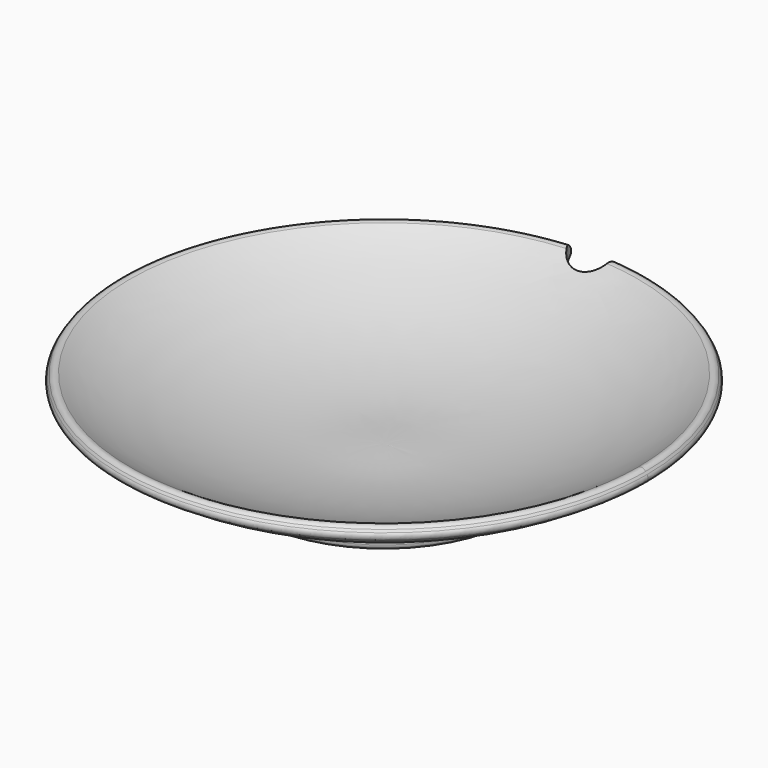
from build123d import *

# Parameters (mm, degrees)
F2_R     = 11.1276169932
F3_DEPTH = 87.884
F4_R     = 64.6620643292
F4_R_2   = 55.3121936168
F5_DEPTH = 5.334
F6_R     = 2.54


# Not quite as in the source:
# - ends of sketch curves that miss each other by under 0.0002 mm in the source are joined
# - the dataset's text gives a spline's control points without its knots; the knots are read off the source's solid


with BuildPart() as f1:
    # F0 (on Front) → F1 (revolve)
    with BuildSketch(Plane.XZ):
        with BuildLine():
            Line((0, 6.35), (0, 0))
            Line((0, 0), (0.2311245356, 0.0031557032))
            add(Edge.make_bspline(
                [(0.2311245356, 0.0031557032), (2.4501256753, 0.0426217254), (7.0028418067, 0.0144777686), (13.0289667294, -0.1317788571), (18.1484598292, -0.2072564384), (22.1362226559, -0.213579989), (25.59517992, -0.152370773), (28.45022654, -0.0488424002), (31.3678886248, 0.0965344282), (35.1049795451, 0.3597888187), (41.2551793589, 0.954186617), (49.2172461824, 2.0237910002), (57.4214862458, 3.5344501339), (64.054003418, 5.012225469), (69.0440735463, 6.2568213064), (74.0295963368, 7.6382335755), (78.9953418837, 9.1618676832), (83.885190459, 10.805825477), (90.2620560642, 13.1212282101), (97.879793262, 16.1837036596), (104.8000199937, 19.3010031818), (109.7839369102, 21.7301391734), (113.2145299778, 23.4965291676), (116.307031409, 25.1873599823), (119.0350420871, 26.7770748613), (121.4643085074, 28.2736101039), (123.6466120059, 29.6781464391), (125.6372412687, 30.9921674342), (126.875727056, 31.8112669996), (127.4840118173, 32.2088484326)],
                knots=[0.0010428138, 0.0010428138, 0.0010428138, 0.0010428138, 0.0625, 0.125, 0.15625, 0.1875, 0.21875, 0.234375, 0.25, 0.28125, 0.3125, 0.375, 0.4375, 0.46875, 0.5, 0.53125, 0.5625, 0.59375, 0.625, 0.6875, 0.75, 0.78125, 0.8125, 0.84375, 0.875, 0.90625, 0.9375, 0.96875, 1, 1, 1, 1], degree=3))
            Line((127.4840118173, 32.2088484326), (124.0098550916, 37.5241786242))
            add(Edge.make_bspline(
                [(0, 6.35), (9.1538715789, 6.5204219784), (29.9872491064, 4.9113894456), (74.2028739049, 12.1904680597), (111.5084892236, 28.9700197615), (120.6347367824, 35.3181651591), (124.0098550916, 37.5241786242)],
                knots=[0, 0, 0, 0, 0.2423270049, 0.5463573209, 0.8319700359, 1, 1, 1, 1], degree=3))
        make_face()
    revolve(axis=Axis((0, 0, 3.175), (0, 0, 1)))

    # F2 (on Top) → F3 (cut)
    with BuildSketch(Plane.XY):
        with Locations((0, 126.9588023424)):
            Circle(F2_R)
    extrude(amount=F3_DEPTH, mode=Mode.SUBTRACT)

    # F4 (on Top) → F5 (join, symmetric)
    with BuildSketch(Plane.XY):
        Circle(F4_R)
        Circle(F4_R_2, mode=Mode.SUBTRACT)
    extrude(amount=F5_DEPTH, both=True)

    # F6
    f6_edges = [f1.edges().sort_by_distance(p)[0] for p in [
        (-64.662064, 0, -5.334),
        (-64.662064, 0, 5.178882),
        (-55.312194, 0, -5.334),
        (-55.312194, 0, 3.170681),
        (93.996697, 86.120812, 32.208848),
        (-86.120812, -93.996697, 32.208848),
        (91.357245, 83.858798, 37.524179),
        (-83.858798, -91.357245, 37.524179),
    ]]
    fillet(f6_edges, radius=F6_R)


solid = f1.part
